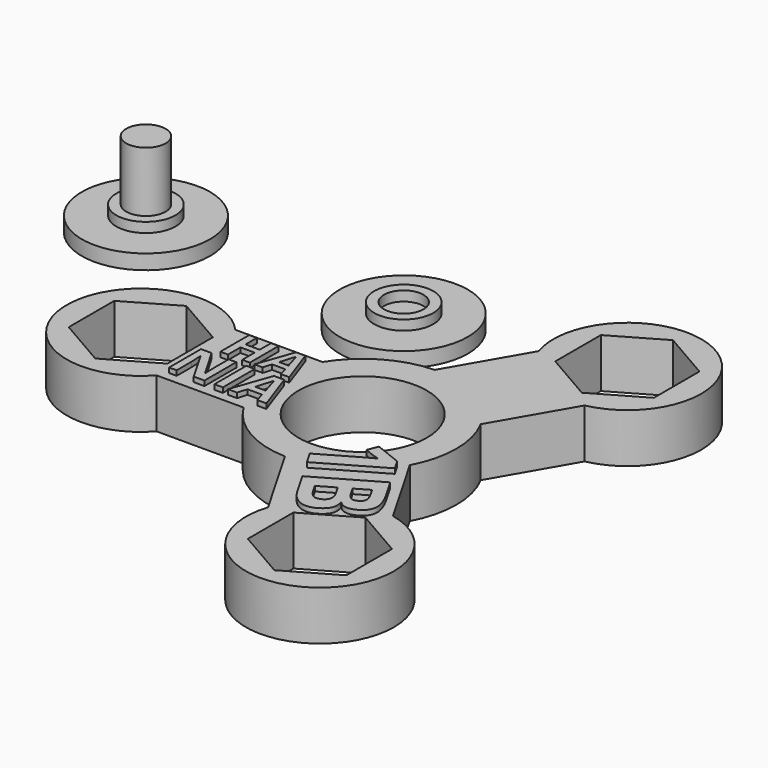
from build123d import *

# Parameters (mm, degrees)
F0_W           = 0.8560095915
F0_H           = 4.036230984
F0_R           = 6.5
F0_TEXT_SIZE   = 9.8641075763
F0_TEXT_SIZE_2 = 5.1150604526
F0_TEXT_SIZE_3 = 5.6537269201
F1_DEPTH       = 5
F2_R           = 6.5
F2_R_2         = 3
F2_R_3         = 2
F3_DEPTH       = 1.5
F4_DEPTH       = 2.5
F5_DEPTH       = 8.6
F6_DEPTH       = 5.5


# Not quite as in the source:
# - Text() gives the source's letters only with a copy of the font that has no kerning and outlines rounded to 1/6400 em; it was checked with that copy


with BuildPart() as f1:
    # F0 (on Top) → F1 (new body)
    with BuildSketch(Plane.XY):
        with BuildLine():
            ThreePointArc((-0.2912534136, 9.4955342898), (-4.75, 8.227241336), (-8.0777472107, 5))
            Line((-8.0777472107, 5), (-16.9098300563, 5))
            ThreePointArc((-16.9098300563, 5), (-30, 0), (-16.9098300563, -5))
            Line((-16.9098300563, -5), (-8.0777472107, -5))
            ThreePointArc((-8.0777472107, -5), (-4.75, -8.227241336), (-0.2912534136, -9.4955342898))
            Line((-0.2912534136, -9.4955342898), (4.1247880092, -17.1443424024))
            ThreePointArc((4.1247880092, -17.1443424024), (15, -25.9807621135), (12.785042047, -12.1443424024))
            Line((12.785042047, -12.1443424024), (8.3690006243, -4.4955342898))
            ThreePointArc((8.3690006243, -4.4955342898), (9.5, 0), (8.3690006243, 4.4955342898))
            Line((8.3690006243, 4.4955342898), (12.785042047, 12.1443424024))
            ThreePointArc((12.785042047, 12.1443424024), (15, 25.9807621135), (4.1247880092, 17.1443424024))
            Line((4.1247880092, 17.1443424024), (-0.2912534136, 9.4955342898))
        make_face()
        with BuildLine():
            Line((-12.7908328925, -0.0344523984), (-12.7908328925, -4.0706833825))
            Line((-12.7908328925, -4.0706833825), (-13.8782919298, -4.0706833825))
            Line((-13.8782919298, -4.0706833825), (-15.6344808543, -1.0176708456))
            Line((-15.6344808543, -1.0176708456), (-15.6592159096, -1.0176708456))
            add(Edge.make_bspline(
                [(-15.6592159096, -1.0176708456), (-15.6062122197, -1.8259771162), (-15.6062122197, -2.1713844952)],
                knots=[0, 0, 0, 1, 1, 1], degree=2))
            Line((-15.6062122197, -2.1713844952), (-15.6062122197, -4.0706833825))
            Line((-15.6062122197, -4.0706833825), (-16.3712321436, -4.0706833825))
            Line((-16.3712321436, -4.0706833825), (-16.3712321436, -0.0344523984))
            Line((-16.3712321436, -0.0344523984), (-15.2917236598, -0.0344523984))
            Line((-15.2917236598, -0.0344523984), (-13.5390683146, -3.057429511))
            Line((-13.5390683146, -3.057429511), (-13.5196336283, -3.057429511))
            add(Edge.make_bspline(
                [(-13.5196336283, -3.057429511), (-13.5611531853, -2.2703247163), (-13.5611531853, -1.9452354184)],
                knots=[0, 0, 0, 1, 1, 1], degree=2))
            Line((-13.5611531853, -1.9452354184), (-13.5611531853, -0.0344523984))
            Line((-13.5611531853, -0.0344523984), (-12.7908328925, -0.0344523984))
        make_face(mode=Mode.SUBTRACT)
        with Locations((-11.3469240408, -2.0525678904)):
            Rectangle(F0_W, F0_H, mode=Mode.SUBTRACT)
        Polygon((-6.5098956422, -4.0706833825), (-7.4321598461, -4.0706833825), (-7.7245635352, -3.109549806), (-9.1962993241, -3.109549806), (-9.4887030132, -4.0706833825), (-10.4109672171, -4.0706833825), (-8.9860513542, -0.0176678966), (-7.940111874, -0.0176678966), align=None, mode=Mode.SUBTRACT)
        Polygon((16.25, -16.5988202392), (16.25, -22.3723229311), (11.25, -25.259074277), (6.25, -22.3723229311), (6.25, -16.5988202392), (11.25, -13.7120688933), align=None, mode=Mode.SUBTRACT)
        with BuildLine():
            Line((8.3857457098, -6.4042755637), (2.2871532043, -9.9252995884))
            Line((2.2871532043, -9.9252995884), (1.5427213357, -8.6359057691))
            Line((1.5427213357, -8.6359057691), (5.071869636, -6.5983510479))
            Line((5.071869636, -6.5983510479), (5.6588688454, -6.2772439125))
            Line((5.6588688454, -6.2772439125), (6.3044470464, -5.9312146885))
            add(Edge.make_bspline(
                [(6.3044470464, -5.9312146885), (5.7991487389, -5.7958204151), (5.6266009831, -5.7281489566)],
                knots=[0, 0, 0, 1, 1, 1], degree=2))
            Line((5.6266009831, -5.7281489566), (4.658742885, -5.3525987428))
            Line((4.658742885, -5.3525987428), (5.0751326968, -4.2828550208))
            Line((5.0751326968, -4.2828550208), (7.7738627867, -5.3444632526))
            Line((7.7738627867, -5.3444632526), (8.3857457098, -6.4042755637))
        make_face(mode=Mode.SUBTRACT)
        with BuildLine():
            Line((3.5078365169, -12.0395851057), (9.6064290223, -8.518561081))
            Line((9.6064290223, -8.518561081), (10.7022697234, -10.4166128522))
            add(Edge.make_bspline(
                [(10.7022697234, -10.4166128522), (11.4513253924, -11.7140153288), (11.4205678348, -12.5130622215)],
                knots=[0, 0, 0, 1, 1, 1], degree=2))
            add(Edge.make_bspline(
                [(11.4205678348, -12.5130622215), (11.3898102771, -13.3121091142), (10.5849402223, -13.776801057)],
                knots=[0, 0, 0, 1, 1, 1], degree=2))
            add(Edge.make_bspline(
                [(10.5849402223, -13.776801057), (10.037681976, -14.0927607528), (9.5393416071, -14.0387749891)],
                knots=[0, 0, 0, 1, 1, 1], degree=2))
            add(Edge.make_bspline(
                [(9.5393416071, -14.0387749891), (9.0410012382, -13.9847892253), (8.7244260431, -13.5998391846)],
                knots=[0, 0, 0, 1, 1, 1], degree=2))
            Line((8.7244260431, -13.5998391846), (8.6830479805, -13.6237288202))
            add(Edge.make_bspline(
                [(8.6830479805, -13.6237288202), (8.8880295856, -14.2777731357), (8.6819934321, -14.7393207251)],
                knots=[0, 0, 0, 1, 1, 1], degree=2))
            add(Edge.make_bspline(
                [(8.6819934321, -14.7393207251), (8.4759572786, -15.2008683145), (7.8873209698, -15.5407176458)],
                knots=[0, 0, 0, 1, 1, 1], degree=2))
            add(Edge.make_bspline(
                [(7.8873209698, -15.5407176458), (7.0530858383, -16.0223635236), (6.2375878658, -15.688766368)],
                knots=[0, 0, 0, 1, 1, 1], degree=2))
            add(Edge.make_bspline(
                [(6.2375878658, -15.688766368), (5.4220898934, -15.3551692124), (4.824849005, -14.3207176493)],
                knots=[0, 0, 0, 1, 1, 1], degree=2))
            Line((4.824849005, -14.3207176493), (3.5078365169, -12.0395851057))
        make_face(mode=Mode.SUBTRACT)
        Polygon((-22.5, -5.7735026919), (-27.5, -2.8867513459), (-27.5, 2.8867513459), (-22.5, 5.7735026919), (-17.5, 2.8867513459), (-17.5, -2.8867513459), align=None, mode=Mode.SUBTRACT)
        Polygon((-11.9010940986, 4.2260180461), (-11.9010940986, 0.5743444199), (-12.6731485357, 0.5743444199), (-12.6731485357, 2.1504224218), (-14.1189523418, 2.1504224218), (-14.1189523418, 0.5743444199), (-14.8934044634, 0.5743444199), (-14.8934044634, 4.2260180461), (-14.1189523418, 4.2260180461), (-14.1189523418, 2.7946003476), (-12.6731485357, 2.7946003476), (-12.6731485357, 4.2260180461), align=None, mode=Mode.SUBTRACT)
        Polygon((-7.9097484892, 0.5743444199), (-8.7441427255, 0.5743444199), (-9.0086872583, 1.4439046968), (-10.3402014324, 1.4439046968), (-10.6047459652, 0.5743444199), (-11.4391402015, 0.5743444199), (-10.1499851218, 4.2412033819), (-9.2036989381, 4.2412033819), align=None, mode=Mode.SUBTRACT)
        Circle(F0_R, mode=Mode.SUBTRACT)
        Polygon((6.25, 22.3723229311), (11.25, 25.259074277), (16.25, 22.3723229311), (16.25, 16.5988202392), (11.25, 13.7120688933), (6.25, 16.5988202392), align=None, mode=Mode.SUBTRACT)
        with BuildLine():
            Line((7.3744997633, -12.5995178717), (6.9121197207, -11.7986521454))
            Line((6.9121197207, -11.7986521454), (5.3224012541, -12.7164765301))
            Line((5.3224012541, -12.7164765301), (5.8086709323, -13.5587203189))
            add(Edge.make_bspline(
                [(5.8086709323, -13.5587203189), (6.116924294, -14.092630803), (6.4679507177, -14.2289987603)],
                knots=[0, 0, 0, 1, 1, 1], degree=2))
            add(Edge.make_bspline(
                [(6.4679507177, -14.2289987603), (6.8189771415, -14.3653667175), (7.240766424, -14.1218465617)],
                knots=[0, 0, 0, 1, 1, 1], degree=2))
            add(Edge.make_bspline(
                [(7.240766424, -14.1218465617), (8.0002540877, -13.6833561546), (7.3744997633, -12.5995178717)],
                knots=[0, 0, 0, 1, 1, 1], degree=2))
        make_face()
        with BuildLine():
            Line((9.2933604801, -10.423842152), (7.9372278503, -11.2068056909))
            Line((7.9372278503, -11.2068056909), (8.3703238236, -11.9569499211))
            add(Edge.make_bspline(
                [(8.3703238236, -11.9569499211), (8.6739533849, -12.482851748), (8.9728128785, -12.6244224738)],
                knots=[0, 0, 0, 1, 1, 1], degree=2))
            add(Edge.make_bspline(
                [(8.9728128785, -12.6244224738), (9.271672372, -12.7659931996), (9.6467444871, -12.549445213)],
                knots=[0, 0, 0, 1, 1, 1], degree=2))
            add(Edge.make_bspline(
                [(9.6467444871, -12.549445213), (9.9977906305, -12.3467686277), (10.0019935048, -12.0026393872)],
                knots=[0, 0, 0, 1, 1, 1], degree=2))
            add(Edge.make_bspline(
                [(10.0019935048, -12.0026393872), (10.0061963792, -11.6585101466), (9.6856128829, -11.1032432431)],
                knots=[0, 0, 0, 1, 1, 1], degree=2))
            Line((9.6856128829, -11.1032432431), (9.2933604801, -10.423842152))
        make_face()
        with Locations(Location((0.2495984831, -6.396151288), (0, 0, -60))):
            Text('1B', F0_TEXT_SIZE, font='Open Sans', font_style=FontStyle.BOLD, text_align=(TextAlign.LEFT, TextAlign.BOTTOM))
        with BuildLine():
            Line((-8.9807509853, -2.3922332031), (-7.9295111361, -2.3922332031))
            add(Edge.make_bspline(
                [(-7.9295111361, -2.3922332031), (-8.3349893636, -1.0865756425), (-8.3862262638, -0.9151970452)],
                knots=[0, 0, 0, 1, 1, 1], degree=2))
            add(Edge.make_bspline(
                [(-8.3862262638, -0.9151970452), (-8.437463164, -0.7438184479), (-8.4595480348, -0.6448782268)],
                knots=[0, 0, 0, 1, 1, 1], degree=2))
            add(Edge.make_bspline(
                [(-8.4595480348, -0.6448782268), (-8.5505377024, -0.9982361593), (-8.9807509853, -2.3922332031)],
                knots=[0, 0, 0, 1, 1, 1], degree=2))
        make_face()
        with BuildLine():
            Line((-10.1451897526, 2.0928779917), (-9.1941081997, 2.0928779917))
            add(Edge.make_bspline(
                [(-9.1941081997, 2.0928779917), (-9.5609539415, 3.274137265), (-9.6073091769, 3.429187535)],
                knots=[0, 0, 0, 1, 1, 1], degree=2))
            add(Edge.make_bspline(
                [(-9.6073091769, 3.429187535), (-9.6536644123, 3.584237805), (-9.6736451171, 3.6737513629)],
                knots=[0, 0, 0, 1, 1, 1], degree=2))
            add(Edge.make_bspline(
                [(-9.6736451171, 3.6737513629), (-9.7559656213, 3.3540600846), (-10.1451897526, 2.0928779917)],
                knots=[0, 0, 0, 1, 1, 1], degree=2))
        make_face()
        with Locations((-15.352960676, 0.5743444199)):
            Text('HA', F0_TEXT_SIZE_2, font='Open Sans', font_style=FontStyle.BOLD, text_align=(TextAlign.LEFT, TextAlign.BOTTOM))
        with Locations((-16.8791841716, -4.0706833825)):
            Text('NIA', F0_TEXT_SIZE_3, font='Open Sans', font_style=FontStyle.BOLD, text_align=(TextAlign.LEFT, TextAlign.BOTTOM))
    extrude(amount=F1_DEPTH)

    # F0 (on Top) → F6 (join)
    with BuildSketch(Plane.XY):
        with Locations((-16.8791841716, -4.0706833825)):
            Text('NIA', F0_TEXT_SIZE_3, font='Open Sans', font_style=FontStyle.BOLD, text_align=(TextAlign.LEFT, TextAlign.BOTTOM))
        with Locations((-15.352960676, 0.5743444199)):
            Text('HA', F0_TEXT_SIZE_2, font='Open Sans', font_style=FontStyle.BOLD, text_align=(TextAlign.LEFT, TextAlign.BOTTOM))
        with Locations(Location((0.2495984831, -6.396151288), (0, 0, -60))):
            Text('1B', F0_TEXT_SIZE, font='Open Sans', font_style=FontStyle.BOLD, text_align=(TextAlign.LEFT, TextAlign.BOTTOM))
    extrude(amount=F6_DEPTH)


with BuildPart() as f3:
    # F2 (on Top) → F3 (new body)
    with BuildSketch(Plane.XY):
        with Locations((-12.4751891814, 20.7975374452)):
            Circle(F2_R)
        with Locations((-12.4751891814, 20.7975374452)):
            Circle(F2_R_2, mode=Mode.SUBTRACT)
        with Locations((-12.4751891814, 20.7975374452)):
            Circle(F2_R_2)
        with Locations((-12.4751891814, 20.7975374452)):
            Circle(F2_R_3, mode=Mode.SUBTRACT)
        with Locations((-12.4751891814, 20.7975374452)):
            Circle(F2_R_3)
    extrude(amount=F3_DEPTH)


with BuildPart() as f3b:
    # F2 (on Top) → F3, piece 2 (new body)
    with BuildSketch(Plane.XY):
        with Locations((-38.877457279, 21.1202766213)):
            Circle(F2_R)
        with Locations((-38.877457279, 21.1202766213)):
            Circle(F2_R_2, mode=Mode.SUBTRACT)
        with Locations((-38.877457279, 21.1202766213)):
            Circle(F2_R_2)
        with Locations((-38.877457279, 21.1202766213)):
            Circle(F2_R_3, mode=Mode.SUBTRACT)
        with Locations((-38.877457279, 21.1202766213)):
            Circle(F2_R_3)
    extrude(amount=F3_DEPTH)


with BuildPart() as f4:
    # F2 (on Top) → F4 (new body)
    with BuildSketch(Plane.XY):
        with Locations((-38.877457279, 21.1202766213)):
            Circle(F2_R_2)
        with Locations((-38.877457279, 21.1202766213)):
            Circle(F2_R_3, mode=Mode.SUBTRACT)
    extrude(amount=F4_DEPTH)


with BuildPart() as f4b:
    # F2 (on Top) → F4, piece 2 (new body)
    with BuildSketch(Plane.XY):
        with Locations((-12.4751891814, 20.7975374452)):
            Circle(F2_R_2)
        with Locations((-12.4751891814, 20.7975374452)):
            Circle(F2_R_3, mode=Mode.SUBTRACT)
    extrude(amount=F4_DEPTH)


with BuildPart() as f5:
    # F2 (on Top) → F5 (new body)
    with BuildSketch(Plane.XY):
        with Locations((-38.877457279, 21.1202766213)):
            Circle(F2_R_3)
    extrude(amount=F5_DEPTH)


solid = Compound([f1.part, f3.part, f3b.part, f4.part, f4b.part, f5.part])
